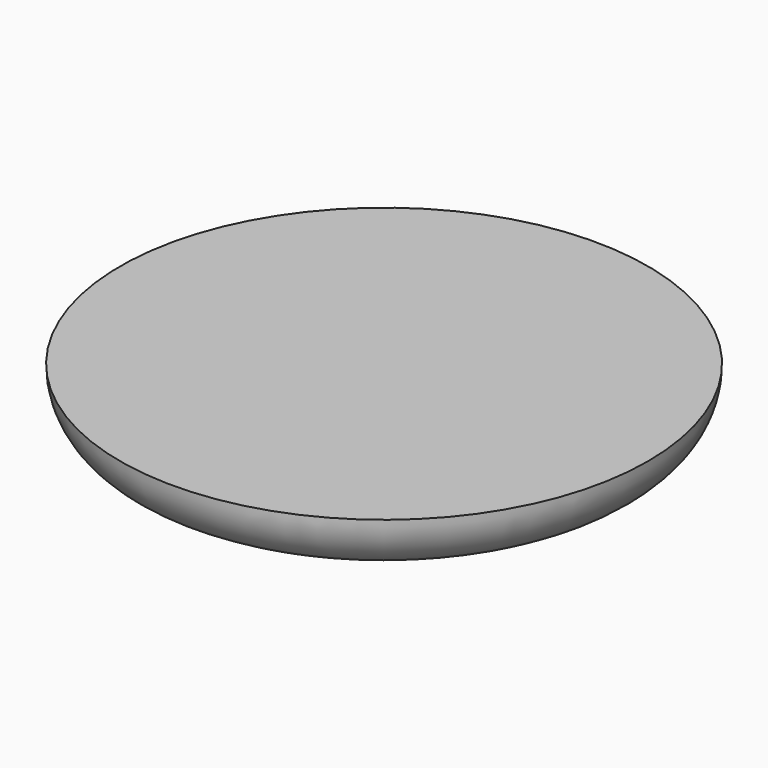
from build123d import *

# Parameters (mm, degrees)
F0_R     = 22.5
F1_DEPTH = 5
F2_R     = 4.99999


# Not quite as in the source:
# - a fillet or chamfer is up to 0.001 mm smaller than in the source, because OpenCascade refuses the exact size


with BuildPart() as f1:
    # F0 (on Top) → F1 (new body)
    with BuildSketch(Plane.XY):
        Circle(F0_R)
    extrude(amount=F1_DEPTH)

    # F2 (radius 5 in the source; OpenCascade refuses exactly that, so slightly less here)
    f2_edges = [f1.edges().sort_by_distance(p)[0] for p in [
        (-22.5, 0, 0),
    ]]
    fillet(f2_edges, radius=F2_R)


solid = f1.part
